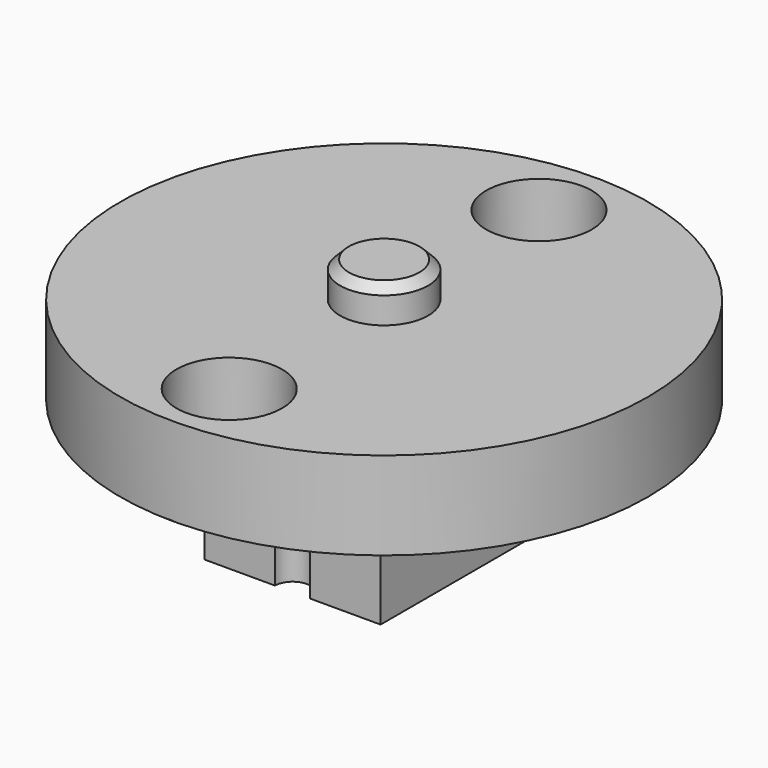
from build123d import *

# Parameters (mm, degrees)
F0_W      = 5
F0_H      = 6.5
F1_DEPTH  = 3.5
F2_R      = 7.5
F2_R_2    = 1.5
F2_W      = 5
F2_H      = 6.5
F3_DEPTH  = 2.5
F4_R      = 1.25
F5_DEPTH  = 1
F6_SIZE   = 0.49999
F7_SIZE   = 0.25
F8_W      = 1
F8_H      = 0.5
F9_DEPTH  = 0.3
F10_R     = 0.5
F11_DEPTH = 3.19


# Not quite as in the source:
# - a fillet or chamfer is up to 0.001 mm smaller than in the source, because OpenCascade refuses the exact size


with BuildPart() as f1:
    # F0 (on Top) → F1 (new body)
    with BuildSketch(Plane.XY):
        Rectangle(F0_W, F0_H)
        Polygon((-0.75, -2), (-0.75, -0.5), (-2.25, -0.5), (-2.25, 0.5), (-0.75, 0.5), (-0.75, 2), (0.75, 2), (0.75, 0.5), (2.25, 0.5), (2.25, -0.5), (0.75, -0.5), (0.75, -2), align=None, mode=Mode.SUBTRACT)
    extrude(amount=F1_DEPTH)

    # F2 (on face) → F3 (join)
    with BuildSketch(Plane.XY.offset(3.5)):
        Circle(F2_R)
        with Locations((0, -5.5)):
            Circle(F2_R_2, mode=Mode.SUBTRACT)
        Rectangle(F2_W, F2_H, mode=Mode.SUBTRACT)
        with Locations((0, 5.5)):
            Circle(F2_R_2, mode=Mode.SUBTRACT)
        Rectangle(F2_W, F2_H)
        Polygon((0.75, -2), (-0.75, -2), (-0.75, -0.5), (-2.25, -0.5), (-2.25, 0.5), (-0.75, 0.5), (-0.75, 2), (0.75, 2), (0.75, 0.5), (2.25, 0.5), (2.25, -0.5), (0.75, -0.5), align=None, mode=Mode.SUBTRACT)
        Polygon((-0.75, -0.5), (-0.75, -2), (0.75, -2), (0.75, -0.5), (2.25, -0.5), (2.25, 0.5), (0.75, 0.5), (0.75, 2), (-0.75, 2), (-0.75, 0.5), (-2.25, 0.5), (-2.25, -0.5), align=None)
    extrude(amount=F3_DEPTH)

    # F4 (on face) → F5 (join)
    with BuildSketch(Plane.XY.offset(6)):
        Circle(F4_R)
    extrude(amount=F5_DEPTH)

    # F6 (size 0.5 in the source; OpenCascade refuses exactly that, so slightly less here)
    f6_edges = [f1.edges().sort_by_distance(p)[0] for p in [
        (-1.5, 5.5, 3.5),
        (-1.5, -5.5, 3.5),
    ]]
    chamfer(f6_edges, length=F6_SIZE)

    # F7
    f7_edges = [f1.edges().sort_by_distance(p)[0] for p in [
        (-1.25, 0, 7),
    ]]
    chamfer(f7_edges, length=F7_SIZE)

    # F8 (on face) → F9 (join)
    with BuildSketch(Plane(origin=(-2.5, 0, 0), x_dir=(0, -1, 0), z_dir=(-1, 0, 0))):
        with Locations((0, 0.75)):
            Rectangle(F8_W, F8_H)
    extrude(amount=-F9_DEPTH)

    # F10 (on face) → F11 (cut)
    with BuildSketch(Plane.XY):
        with Locations((0, -3.25)):
            Circle(F10_R)
    extrude(amount=F11_DEPTH, mode=Mode.SUBTRACT)


solid = f1.part
